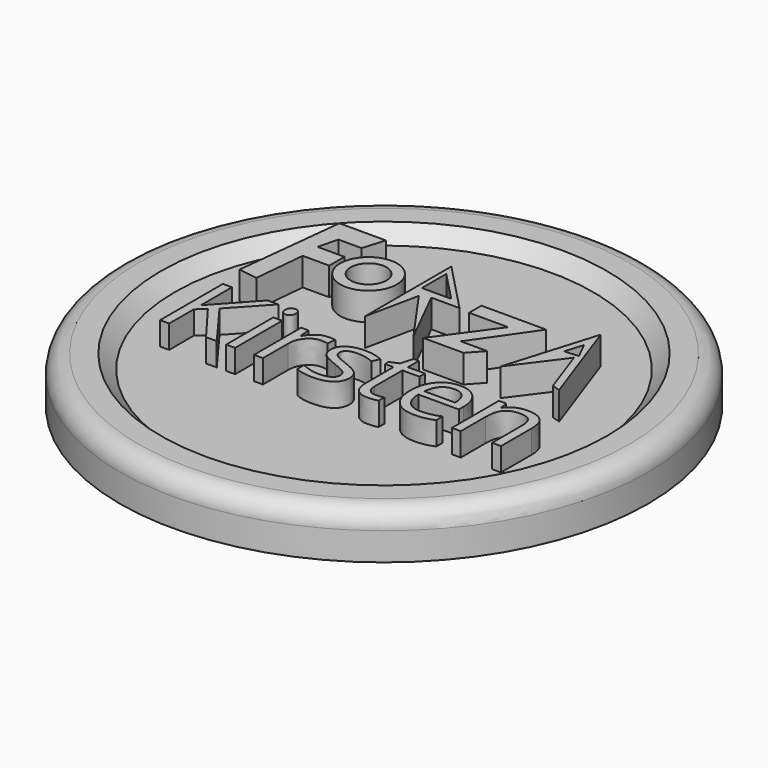
from build123d import *

# Parameters (mm, degrees)
F0_R         = 55.9427564204
F1_DEPTH     = 8.89
F0_R_2       = 72.2340030235
F2_DEPTH     = 12.7
F4_R         = 5.08
F5_R         = 7.7731283097
F5_R_2       = 4.9007638307
F6_DEPTH     = 7.62
F7_TEXT_SIZE = 30.0662152262
F8_DEPTH     = 6.35
F9_R         = 14.3615021741
F9_R_2       = 9.7131370875
F10_DEPTH    = 7.62
F12_W        = 29.9027264118
F12_H        = 15.0860603899
F13_DEPTH    = 25.4


# Not quite as in the source:
# - a fillet or chamfer that OpenCascade refuses, or shapes differently, is made with other operations: its cross-section is extruded or revolved along the edge and cut away or added
# - Text() gives the source's letters only with a copy of the font that has no kerning and outlines rounded to 1/6400 em; it was checked with that copy


with BuildPart() as f1:
    # F0 (on Top) → F1 (new body)
    with BuildSketch(Plane.XY):
        Circle(F0_R)
    extrude(amount=F1_DEPTH)

    # F0 (on Top) → F2 (join)
    with BuildSketch(Plane.XY):
        Circle(F0_R_2)
        Circle(F0_R, mode=Mode.SUBTRACT)
    extrude(amount=F2_DEPTH)

    # F3: chamfer of 5.08 on 1 edges, made by hand


with BuildPart() as f3_tool2:
    # F3_s3 → F3_t4 (revolve)
    with BuildSketch(Plane.XZ):
        Polygon((61.0227564204, 12.7), (55.9427564204, 7.62), (55.9427564204, 12.7), align=None)
    revolve(axis=Axis((0, 0, 12.7), (0, 0, 1)))

    split(bisect_by=Plane.XY.offset(8.89), keep=Keep.TOP)


with BuildPart() as f1_1:
    add(f1.part)

    # F3_t1: cut F3_tool2
    add(f3_tool2.part, mode=Mode.SUBTRACT)

    # F4
    f4_edges = [f1_1.edges().sort_by_distance(p)[0] for p in [
        (-72.234003, 0, 12.7),
    ]]
    fillet(f4_edges, radius=F4_R)

    # F5 (on face) → F6 (join)
    with BuildSketch(Plane.XY.offset(8.89)):
        Polygon((-40.4827147722, 35.3630334139), (-43.7674373388, 5.3450884297), (-38.557190448, 4.552161321), (-37.1979959309, 18.7115706503), (-29.9489591271, 18.7115706503), (-29.9489591271, 23.922232911), (-37.3112633824, 23.922232911), (-35.9520688653, 29.3594449759), (-29.6091604978, 29.3594449759), (-27.7969017625, 35.3630334139), align=None)
        with Locations((-21.0009291768, 20.9770742804)):
            Circle(F5_R)
        with Locations((-21.0009291768, 20.9770742804)):
            Circle(F5_R_2, mode=Mode.SUBTRACT)
        Polygon((-9.3326754868, 34.6975848079), (-9.3326754868, 5.1327394322), (-6.2744882889, 19.7452493012), (4.4858003967, 4.4530876912), (-3.6693664733, 20.7647271454), (4.0327357128, 20.7647271454), align=None)
        Polygon((-8.0253826454, 22.9828748852), (-8.0253826454, 31.3130356371), (0, 22.9828748852), align=None, mode=Mode.SUBTRACT)
        Polygon((6.6167367622, 5.1327394322), (17.6651775837, 5.1327394322), (21.0940018296, 8.9207049459), (13.8553734869, 8.9207049459), (24.7133169323, 24.5421603322), (6.9977170788, 24.5421603322), (6.9977170788, 20.3510373831), (17.6651775837, 20.3510373831), align=None)
        Polygon((35.2687533918, 30.0036323336), (27.7611613274, 5.1327394322), (37.470772254, 18.1306428082), (42.082292377, 5.1327394322), (44.3338192999, 4.4530876912), align=None)
        Polygon((37.8195128803, 19.3664522198), (33.9947976172, 19.0732423216), (35.4898783309, 24.0260943135), align=None, mode=Mode.SUBTRACT)
    extrude(amount=F6_DEPTH)

    # F7 (on face) → F8 (join)
    with BuildSketch(Plane.XY.offset(8.89)):
        with Locations((-46.8775179975, -21.6476749629)):
            Text('Kirsten', F7_TEXT_SIZE, font='Open Sans', text_align=(TextAlign.LEFT, TextAlign.BOTTOM))
    extrude(amount=F8_DEPTH)


with BuildPart() as f10:
    # F9 (on Front) → F10 (new body)
    with BuildSketch(Plane.XZ):
        with Locations((-31.1150010675, -18.1840918958)):
            Circle(F9_R)
        with Locations((-31.1150010675, -18.1840918958)):
            Circle(F9_R_2, mode=Mode.SUBTRACT)
    extrude(amount=F10_DEPTH)

    # F11: fillet of radius 5.08 on 1 edges, made by hand

    # F11_s1 → F11_t2 (revolve, cut)
    with BuildSketch(Plane.XY.offset(-18.1840918958)):
        with BuildLine():
            ThreePointArc((-16.7530988934, -2.5574839241), (-18.0915611523, -5.9941903661), (-21.4018299234, -7.6203985476))
            Line((-21.4018299234, -7.6203985476), (-21.3585664579, -8.1266900099))
            ThreePointArc((-21.3585664579, -8.1266900099), (-19.0776644084, -8.1281365685), (-16.7534988934, -8.1281365685))
            Line((-16.7534988934, -8.1281365685), (-16.2453623248, -7.62))
            ThreePointArc((-16.2453623248, -7.62), (-16.2453623248, -5.0887419621), (-16.2449623248, -2.5574839241))
            Line((-16.2449623248, -2.5574839241), (-16.7530988934, -2.5574839241))
        make_face()
    revolve(axis=Axis((-31.1150010675, -7.62, -18.1840918958), (0, -1, 0)), mode=Mode.SUBTRACT)


with BuildPart() as f13:
    # F12 (on Right) → F13 (new body)
    with BuildSketch(Plane.YZ):
        with Locations((35.8293913305, -22.7637877688)):
            Rectangle(F12_W, F12_H)
    extrude(amount=F13_DEPTH)


solid = Compound([f1_1.part, f10.part, f13.part])
